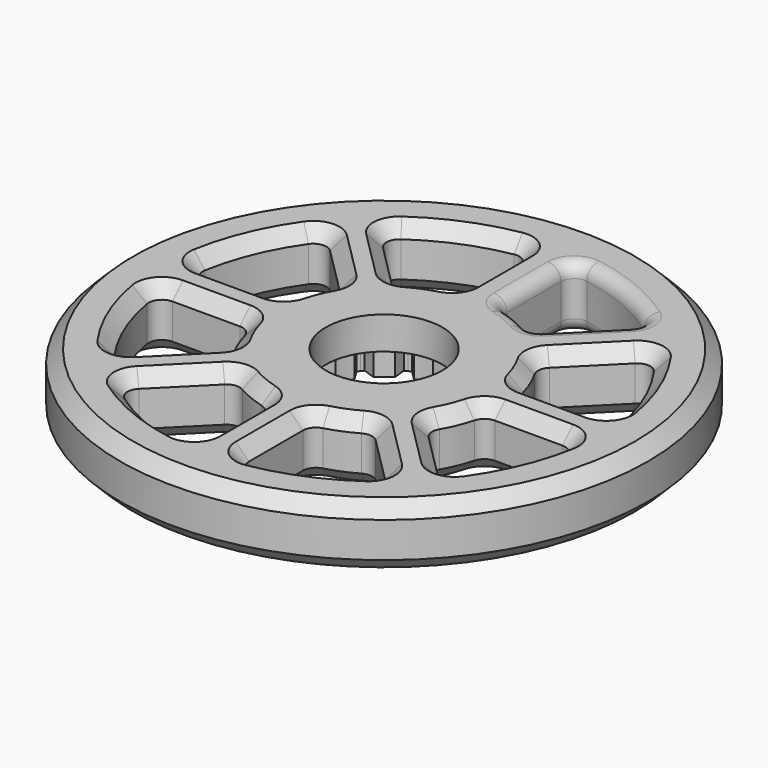
from build123d import *

# Parameters (mm, degrees)
F0_R     = 100
F0_R_2   = 22.1
F1_DEPTH = 23.4
F2_R     = 22.1
F3_DEPTH = 11
F5_DEPTH = 25
F6_F1_R  = 5
F6_F2_R  = 5
F7_SIZE  = 5


with BuildPart() as f1:
    # F0 (on Top) → F1 (new body)
    with BuildSketch(Plane.XY):
        Circle(F0_R)
        Circle(F0_R_2, mode=Mode.SUBTRACT)
    extrude(amount=F1_DEPTH)

    # F2 (on face) → F3 (cut)
    with BuildSketch(Plane(origin=(0, 0, 0), x_dir=(1, 0, 0), z_dir=(0, 0, -1))):
        with BuildLine():
            Line((1.25, -31.4751886412), (2.9, -26.8438074796))
            ThreePointArc((2.9, -26.8438074796), (6.0080652168, -26.3230536289), (9.0342818445, -25.4436976785))
            Line((9.0342818445, -25.4436976785), (12.5303614522, -28.900519751))
            Line((12.5303614522, -28.900519751), (13.6673377822, -28.3805193389))
            Line((13.6673377822, -28.3805193389), (14.782783622, -27.8158104032))
            Line((14.782783622, -27.8158104032), (14.2599012783, -22.9271719916))
            ThreePointArc((14.2599012783, -22.9271719916), (16.8342246502, -21.1094500266), (19.1792133714, -19.0041515057))
            Line((19.1792133714, -19.0041515057), (23.828931144, -20.6017484825))
            Line((23.828931144, -20.6017484825), (24.6276916977, -19.6399287586))
            Line((24.6276916977, -19.6399287586), (25.3876556486, -18.6471697763))
            Line((25.3876556486, -18.6471697763), (22.7954542222, -14.4695289074))
            ThreePointArc((22.7954542222, -14.4695289074), (24.3261594334, -11.7148609562), (25.5254664726, -8.8006000566))
            Line((25.5254664726, -8.8006000566), (30.4078887801, -8.2225482631))
            Line((30.4078887801, -8.2225482631), (30.7102292337, -7.0094094196))
            Line((30.7102292337, -7.0094094196), (30.964191115, -5.7852284827))
            Line((30.964191115, -5.7852284827), (26.8160878895, -3.146018166))
            ThreePointArc((26.8160878895, -3.146018166), (27, 0), (26.8160878895, 3.146018166))
            Line((26.8160878895, 3.146018166), (30.964191115, 5.7852284827))
            Line((30.964191115, 5.7852284827), (30.7102292337, 7.0094094196))
            Line((30.7102292337, 7.0094094196), (30.4078887801, 8.2225482631))
            Line((30.4078887801, 8.2225482631), (25.5254664726, 8.8006000566))
            ThreePointArc((25.5254664726, 8.8006000566), (24.3261594334, 11.7148609562), (22.7954542222, 14.4695289074))
            Line((22.7954542222, 14.4695289074), (25.3876556486, 18.6471697763))
            Line((25.3876556486, 18.6471697763), (24.6276916977, 19.6399287586))
            Line((24.6276916977, 19.6399287586), (23.828931144, 20.6017484825))
            Line((23.828931144, 20.6017484825), (19.1792133714, 19.0041515057))
            ThreePointArc((19.1792133714, 19.0041515057), (16.8342246502, 21.1094500266), (14.2599012783, 22.9271719916))
            Line((14.2599012783, 22.9271719916), (14.782783622, 27.8158104032))
            Line((14.782783622, 27.8158104032), (13.6673377822, 28.3805193389))
            Line((13.6673377822, 28.3805193389), (12.5303614522, 28.900519751))
            Line((12.5303614522, 28.900519751), (9.0342818445, 25.4436976785))
            ThreePointArc((9.0342818445, 25.4436976785), (6.0080652168, 26.3230536289), (2.9, 26.8438074796))
            Line((2.9, 26.8438074796), (1.25, 31.4751886412))
            Line((1.25, 31.4751886412), (0, 31.5))
            Line((0, 31.5), (-1.25, 31.4751886412))
            Line((-1.25, 31.4751886412), (-2.9, 26.8438074796))
            ThreePointArc((-2.9, 26.8438074796), (-6.0080652168, 26.3230536289), (-9.0342818445, 25.4436976785))
            Line((-9.0342818445, 25.4436976785), (-12.5303614522, 28.900519751))
            Line((-12.5303614522, 28.900519751), (-13.6673377822, 28.3805193389))
            Line((-13.6673377822, 28.3805193389), (-14.782783622, 27.8158104032))
            Line((-14.782783622, 27.8158104032), (-14.2599012783, 22.9271719916))
            ThreePointArc((-14.2599012783, 22.9271719916), (-16.8342246502, 21.1094500266), (-19.1792133714, 19.0041515057))
            Line((-19.1792133714, 19.0041515057), (-23.828931144, 20.6017484825))
            Line((-23.828931144, 20.6017484825), (-24.6276916977, 19.6399287586))
            Line((-24.6276916977, 19.6399287586), (-25.3876556486, 18.6471697763))
            Line((-25.3876556486, 18.6471697763), (-22.7954542222, 14.4695289074))
            ThreePointArc((-22.7954542222, 14.4695289074), (-24.3261594334, 11.7148609562), (-25.5254664726, 8.8006000566))
            Line((-25.5254664726, 8.8006000566), (-30.4078887801, 8.2225482631))
            Line((-30.4078887801, 8.2225482631), (-30.7102292337, 7.0094094196))
            Line((-30.7102292337, 7.0094094196), (-30.964191115, 5.7852284827))
            Line((-30.964191115, 5.7852284827), (-26.8160878895, 3.146018166))
            ThreePointArc((-26.8160878895, 3.146018166), (-27, 0), (-26.8160878895, -3.146018166))
            Line((-26.8160878895, -3.146018166), (-30.964191115, -5.7852284827))
            Line((-30.964191115, -5.7852284827), (-30.7102292337, -7.0094094196))
            Line((-30.7102292337, -7.0094094196), (-30.4078887801, -8.2225482631))
            Line((-30.4078887801, -8.2225482631), (-25.5254664726, -8.8006000566))
            ThreePointArc((-25.5254664726, -8.8006000566), (-24.3261594334, -11.7148609562), (-22.7954542222, -14.4695289074))
            Line((-22.7954542222, -14.4695289074), (-25.3876556486, -18.6471697763))
            Line((-25.3876556486, -18.6471697763), (-24.6276916977, -19.6399287586))
            Line((-24.6276916977, -19.6399287586), (-23.828931144, -20.6017484825))
            Line((-23.828931144, -20.6017484825), (-19.1792133714, -19.0041515057))
            ThreePointArc((-19.1792133714, -19.0041515057), (-16.8342246502, -21.1094500266), (-14.2599012783, -22.9271719916))
            Line((-14.2599012783, -22.9271719916), (-14.782783622, -27.8158104032))
            Line((-14.782783622, -27.8158104032), (-13.6673377822, -28.3805193389))
            Line((-13.6673377822, -28.3805193389), (-12.5303614522, -28.900519751))
            Line((-12.5303614522, -28.900519751), (-9.0342818445, -25.4436976785))
            ThreePointArc((-9.0342818445, -25.4436976785), (-6.0080652168, -26.3230536289), (-2.9, -26.8438074796))
            Line((-2.9, -26.8438074796), (-1.25, -31.4751886412))
            Line((-1.25, -31.4751886412), (0, -31.5))
            Line((0, -31.5), (1.25, -31.4751886412))
        make_face()
        Circle(F2_R, mode=Mode.SUBTRACT)
        with BuildLine():
            ThreePointArc((0, -31.5), (0.6251231086, -31.4937965495), (1.25, -31.4751886412))
            Line((1.25, -31.4751886412), (0, -31.5))
        make_face()
        with BuildLine():
            Line((13.6673377822, -28.3805193389), (12.5303614522, -28.900519751))
            ThreePointArc((12.5303614522, -28.900519751), (13.1014297465, -28.6461609749), (13.6673377822, -28.3805193389))
        make_face()
        with BuildLine():
            Line((14.782783622, -27.8158104032), (13.6673377822, -28.3805193389))
            ThreePointArc((13.6673377822, -28.3805193389), (14.2278626653, -28.1036994714), (14.782783622, -27.8158104032))
        make_face()
        with BuildLine():
            ThreePointArc((-13.6673377822, -28.3805193389), (-13.1014297465, -28.6461609749), (-12.5303614522, -28.900519751))
            Line((-12.5303614522, -28.900519751), (-13.6673377822, -28.3805193389))
        make_face()
        with BuildLine():
            Line((24.6276916977, -19.6399287586), (23.828931144, -20.6017484825))
            ThreePointArc((23.828931144, -20.6017484825), (24.2330837617, -20.1248018971), (24.6276916977, -19.6399287586))
        make_face()
        with BuildLine():
            ThreePointArc((-14.782783622, -27.8158104032), (-14.2278626653, -28.1036994714), (-13.6673377822, -28.3805193389))
            Line((-13.6673377822, -28.3805193389), (-14.782783622, -27.8158104032))
        make_face()
        with BuildLine():
            Line((25.3876556486, -18.6471697763), (24.6276916977, -19.6399287586))
            ThreePointArc((24.6276916977, -19.6399287586), (25.0125995279, -19.1473200437), (25.3876556486, -18.6471697763))
        make_face()
        with BuildLine():
            Line((30.7102292337, -7.0094094196), (30.4078887801, -8.2225482631))
            ThreePointArc((30.4078887801, -8.2225482631), (30.5650783387, -7.6174789891), (30.7102292337, -7.0094094196))
        make_face()
        with BuildLine():
            ThreePointArc((-25.3876556486, -18.6471697763), (-25.0125995279, -19.1473200437), (-24.6276916977, -19.6399287586))
            Line((-24.6276916977, -19.6399287586), (-25.3876556486, -18.6471697763))
        make_face()
        with BuildLine():
            Line((30.964191115, -5.7852284827), (30.7102292337, -7.0094094196))
            ThreePointArc((30.7102292337, -7.0094094196), (30.8432842946, -6.3985790549), (30.964191115, -5.7852284827))
        make_face()
        with BuildLine():
            Line((30.7102292337, 7.0094094196), (30.964191115, 5.7852284827))
            ThreePointArc((30.964191115, 5.7852284827), (30.8432842946, 6.3985790549), (30.7102292337, 7.0094094196))
        make_face()
        with BuildLine():
            ThreePointArc((-30.964191115, -5.7852284827), (-30.8432842946, -6.3985790549), (-30.7102292337, -7.0094094196))
            Line((-30.7102292337, -7.0094094196), (-30.964191115, -5.7852284827))
        make_face()
        with BuildLine():
            Line((30.4078887801, 8.2225482631), (30.7102292337, 7.0094094196))
            ThreePointArc((30.7102292337, 7.0094094196), (30.5650783387, 7.6174789891), (30.4078887801, 8.2225482631))
        make_face()
        with BuildLine():
            ThreePointArc((-30.7102292337, 7.0094094196), (-30.8432842946, 6.3985790549), (-30.964191115, 5.7852284827))
            Line((-30.964191115, 5.7852284827), (-30.7102292337, 7.0094094196))
        make_face()
        with BuildLine():
            Line((24.6276916977, 19.6399287586), (25.3876556486, 18.6471697763))
            ThreePointArc((25.3876556486, 18.6471697763), (25.0125995279, 19.1473200437), (24.6276916977, 19.6399287586))
        make_face()
        with BuildLine():
            ThreePointArc((-30.4078887801, 8.2225482631), (-30.5650783387, 7.6174789891), (-30.7102292337, 7.0094094196))
            Line((-30.7102292337, 7.0094094196), (-30.4078887801, 8.2225482631))
        make_face()
        with BuildLine():
            Line((23.828931144, 20.6017484825), (24.6276916977, 19.6399287586))
            ThreePointArc((24.6276916977, 19.6399287586), (24.2330837617, 20.1248018971), (23.828931144, 20.6017484825))
        make_face()
        with BuildLine():
            ThreePointArc((-24.6276916977, 19.6399287586), (-25.0125995279, 19.1473200437), (-25.3876556486, 18.6471697763))
            Line((-25.3876556486, 18.6471697763), (-24.6276916977, 19.6399287586))
        make_face()
        with BuildLine():
            Line((13.6673377822, 28.3805193389), (14.782783622, 27.8158104032))
            ThreePointArc((14.782783622, 27.8158104032), (14.2278626653, 28.1036994714), (13.6673377822, 28.3805193389))
        make_face()
        with BuildLine():
            ThreePointArc((-23.828931144, 20.6017484825), (-24.2330837617, 20.1248018971), (-24.6276916977, 19.6399287586))
            Line((-24.6276916977, 19.6399287586), (-23.828931144, 20.6017484825))
        make_face()
        with BuildLine():
            Line((12.5303614522, 28.900519751), (13.6673377822, 28.3805193389))
            ThreePointArc((13.6673377822, 28.3805193389), (13.1014297465, 28.6461609749), (12.5303614522, 28.900519751))
        make_face()
        with BuildLine():
            ThreePointArc((-13.6673377822, 28.3805193389), (-14.2278626653, 28.1036994714), (-14.782783622, 27.8158104032))
            Line((-14.782783622, 27.8158104032), (-13.6673377822, 28.3805193389))
        make_face()
        with BuildLine():
            Line((0, 31.5), (1.25, 31.4751886412))
            ThreePointArc((1.25, 31.4751886412), (0.6251231086, 31.4937965495), (0, 31.5))
        make_face()
        with BuildLine():
            ThreePointArc((-12.5303614522, 28.900519751), (-13.1014297465, 28.6461609749), (-13.6673377822, 28.3805193389))
            Line((-13.6673377822, 28.3805193389), (-12.5303614522, 28.900519751))
        make_face()
        with BuildLine():
            Line((-1.25, 31.4751886412), (0, 31.5))
            ThreePointArc((0, 31.5), (-0.6251231086, 31.4937965495), (-1.25, 31.4751886412))
        make_face()
    extrude(amount=-F3_DEPTH, mode=Mode.SUBTRACT)

    # F4 (on face) → F5 (cut)
    with BuildSketch(Plane(origin=(0, 0, 0), x_dir=(1, 0, 0), z_dir=(0, 0, -1))):
        with BuildLine():
            ThreePointArc((-44.3044756187, 7.881208039), (-41.574578963, 17.2207544564), (-36.9008507952, 25.7551394985))
            Line((-36.9008507952, 25.7551394985), (-61.8662236407, 50.720512344))
            ThreePointArc((-61.8662236407, 50.720512344), (-73.9103626009, 30.6146745892), (-79.6108444865, 7.881208039))
            Line((-79.6108444865, 7.881208039), (-44.3044756187, 7.881208039))
        make_face()
        with BuildLine():
            Line((-7.881208039, 44.3044756187), (-7.881208039, 79.6108444865))
            ThreePointArc((-7.881208039, 79.6108444865), (-30.6146745892, 73.9103626009), (-50.720512344, 61.8662236407))
            Line((-50.720512344, 61.8662236407), (-25.7551394985, 36.9008507952))
            ThreePointArc((-25.7551394985, 36.9008507952), (-17.2207544564, 41.574578963), (-7.881208039, 44.3044756187))
        make_face()
        with BuildLine():
            ThreePointArc((50.720512344, 61.8662236407), (30.6146745892, 73.9103626009), (7.881208039, 79.6108444865))
            Line((7.881208039, 79.6108444865), (7.881208039, 44.3044756187))
            ThreePointArc((7.881208039, 44.3044756187), (17.2207544564, 41.574578963), (25.7551394985, 36.9008507952))
            Line((25.7551394985, 36.9008507952), (50.720512344, 61.8662236407))
        make_face()
        with BuildLine():
            Line((44.3044756187, 7.881208039), (79.6108444865, 7.881208039))
            ThreePointArc((79.6108444865, 7.881208039), (73.9103626009, 30.6146745892), (61.8662236407, 50.720512344))
            Line((61.8662236407, 50.720512344), (36.9008507952, 25.7551394985))
            ThreePointArc((36.9008507952, 25.7551394985), (41.574578963, 17.2207544564), (44.3044756187, 7.881208039))
        make_face()
        with BuildLine():
            Line((36.9008507952, -25.7551394985), (61.8662236407, -50.720512344))
            ThreePointArc((61.8662236407, -50.720512344), (73.9103626009, -30.6146745892), (79.6108444865, -7.881208039))
            Line((79.6108444865, -7.881208039), (44.3044756187, -7.881208039))
            ThreePointArc((44.3044756187, -7.881208039), (41.574578963, -17.2207544564), (36.9008507952, -25.7551394985))
        make_face()
        with BuildLine():
            Line((7.881208039, -44.3044756187), (7.881208039, -79.6108444865))
            ThreePointArc((7.881208039, -79.6108444865), (30.6146745892, -73.9103626009), (50.720512344, -61.8662236407))
            Line((50.720512344, -61.8662236407), (25.7551394985, -36.9008507952))
            ThreePointArc((25.7551394985, -36.9008507952), (17.2207544564, -41.574578963), (7.881208039, -44.3044756187))
        make_face()
        with BuildLine():
            Line((-25.7551394985, -36.9008507952), (-50.720512344, -61.8662236407))
            ThreePointArc((-50.720512344, -61.8662236407), (-30.6146745892, -73.9103626009), (-7.881208039, -79.6108444865))
            Line((-7.881208039, -79.6108444865), (-7.881208039, -44.3044756187))
            ThreePointArc((-7.881208039, -44.3044756187), (-17.2207544564, -41.574578963), (-25.7551394985, -36.9008507952))
        make_face()
        with BuildLine():
            Line((-44.3044756187, -7.881208039), (-79.6108444865, -7.881208039))
            ThreePointArc((-79.6108444865, -7.881208039), (-73.9103626009, -30.6146745892), (-61.8662236407, -50.720512344))
            Line((-61.8662236407, -50.720512344), (-36.9008507952, -25.7551394985))
            ThreePointArc((-36.9008507952, -25.7551394985), (-41.574578963, -17.2207544564), (-44.3044756187, -7.881208039))
        make_face()
    extrude(amount=-F5_DEPTH, mode=Mode.SUBTRACT)

    # F6: fillet of radius 5 on 34 edges, made by hand

    # F6_f1
    f6_f1_edges = [f1.edges().sort_by_distance(p)[0] for p in [
        (-61.8662236407, -50.720512344, 11.7),
        (-50.720512344, -61.8662236407, 11.7),
        (-36.9008507952, -25.7551394985, 11.7),
        (-7.881208039, -44.3044756187, 11.7),
        (-44.3044756187, -7.881208039, 11.7),
        (25.7551394985, -36.9008507952, 11.7),
        (50.720512344, 61.8662236407, 11.7),
        (-36.9008507952, 25.7551394985, 11.7),
        (-7.881208039, 44.3044756187, 11.7),
        (-44.3044756187, 7.881208039, 11.7),
        (-25.7551394985, 36.9008507952, 11.7),
        (7.881208039, 44.3044756187, 11.7),
        (25.7551394985, 36.9008507952, 11.7),
        (36.9008507952, 25.7551394985, 11.7),
        (44.3044756187, 7.881208039, 11.7),
        (44.3044756187, -7.881208039, 11.7),
        (36.9008507952, -25.7551394985, 11.7),
        (7.881208039, -44.3044756187, 11.7),
        (-25.7551394985, -36.9008507952, 11.7),
        (61.8662236407, 50.720512344, 11.7),
        (7.881208039, 79.6108444865, 11.7),
        (-7.881208039, 79.6108444865, 11.7),
        (-50.720512344, 61.8662236407, 11.7),
        (-61.8662236407, 50.720512344, 11.7),
        (-79.6108444865, 7.881208039, 11.7),
        (-79.6108444865, -7.881208039, 11.7),
        (-7.881208039, -79.6108444865, 11.7),
        (7.881208039, -79.6108444865, 11.7),
        (50.720512344, -61.8662236407, 11.7),
        (61.8662236407, -50.720512344, 11.7),
        (79.6108444865, -7.881208039, 11.7),
        (79.6108444865, 7.881208039, 11.7),
    ]]
    fillet(f6_f1_edges, radius=F6_F1_R)

    # F6_f2
    f6_f2_edges = [f1.edges().sort_by_distance(p)[0] for p in [
        (30.6146745892, 73.9103626009, 0),
        (30.6146745892, 73.9103626009, 23.4),
        (9.6635797209, 77.7126725489, 23.4),
        (48.1179749923, 61.7843404947, 23.4),
        (9.6635797209, 77.7126725489, 0),
        (48.1179749923, 61.7843404947, 0),
    ]]
    fillet(f6_f2_edges, radius=F6_F2_R)

    # F7
    f7_edges = [f1.edges().sort_by_distance(p)[0] for p in [
        (-100, 0, 23.4),
        (-100, 0, 0),
        (-30.614675, 73.910363, 0),
        (-73.910363, 30.614675, 0),
        (-78.811253, 13.739955, 11.7),
        (-65.443587, 46.012356, 11.7),
        (-73.910363, 30.614675, 23.4),
        (-46.012356, 65.443587, 11.7),
        (-13.739955, 78.811253, 11.7),
        (-30.614675, 73.910363, 23.4),
        (-73.910363, -30.614675, 0),
        (-65.443587, -46.012356, 11.7),
        (-78.811253, -13.739955, 11.7),
        (-73.910363, -30.614675, 23.4),
        (-30.614675, -73.910363, 0),
        (-13.739955, -78.811253, 11.7),
        (-46.012356, -65.443587, 11.7),
        (-30.614675, -73.910363, 23.4),
        (30.614675, -73.910363, 0),
        (46.012356, -65.443587, 11.7),
        (13.739955, -78.811253, 11.7),
        (30.614675, -73.910363, 23.4),
        (48.776306, -37.630594, 0),
        (57.817829, -46.672118, 11.7),
        (39.734782, -28.589071, 11.7),
        (48.776306, -37.630594, 23.4),
        (48.776306, 37.630594, 23.4),
        (48.776306, 37.630594, 0),
        (39.734782, 28.589071, 11.7),
        (57.817829, 46.672118, 11.7),
    ]]
    chamfer(f7_edges, length=F7_SIZE)


solid = f1.part
